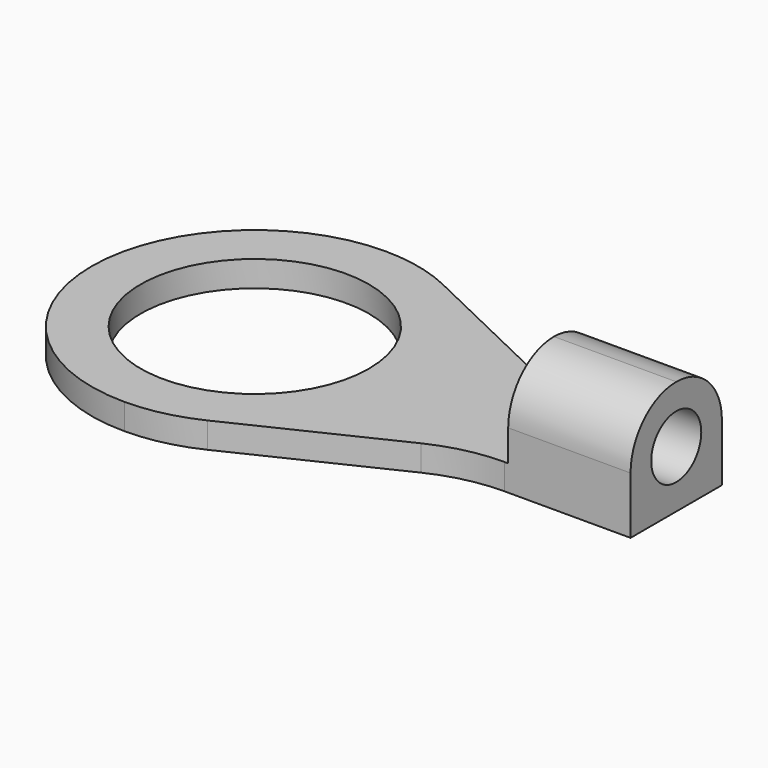
from build123d import *

# Parameters (mm, degrees)
F0_R     = 4.2
F1_DEPTH = 0.95
F2_W     = 4.5
F2_H     = 4.2
F3_DEPTH = 3.25
F4_R     = 2.09999
F5_R     = 1.15
F6_DEPTH = 25


# Not quite as in the source:
# - a fillet or chamfer is up to 0.001 mm smaller than in the source, because OpenCascade refuses the exact size


with BuildPart() as f1:
    # F0 (on Top) → F1 (new body)
    with BuildSketch(Plane.XY):
        with BuildLine():
            Line((16.8637172922, 3.9), (21.5, 3.9))
            Line((21.5, 3.9), (21.5, 8.1))
            Line((21.5, 8.1), (16.8637172922, 8.1))
            ThreePointArc((16.8637172922, 8.1), (15.5339156309, 8.2492199202), (14.2702582689, 8.6894574861))
            Line((14.2702582689, 8.6894574861), (8.5934590232, 11.4105425139))
            ThreePointArc((8.5934590232, 11.4105425139), (7.3298016613, 11.8507800798), (6, 12))
            ThreePointArc((6, 12), (1.7573593129, 10.2426406871), (0, 6))
            ThreePointArc((0, 6), (1.7573593129, 1.7573593129), (6, 0))
            ThreePointArc((6, 0), (7.3298016613, 0.1492199202), (8.5934590232, 0.5894574861))
            Line((8.5934590232, 0.5894574861), (14.2702582689, 3.3105425139))
            ThreePointArc((14.2702582689, 3.3105425139), (15.5339156309, 3.7507800798), (16.8637172922, 3.9))
        make_face()
        with Locations((6, 6)):
            Circle(F0_R, mode=Mode.SUBTRACT)
    extrude(amount=F1_DEPTH)

    # F2 (on face) → F3 (join)
    with BuildSketch(Plane.XY.offset(0.95)):
        with Locations((19.25, 6)):
            Rectangle(F2_W, F2_H)
    extrude(amount=F3_DEPTH)

    # F4 (radius 2.1 in the source; OpenCascade refuses exactly that, so slightly less here)
    f4_edges = [f1.edges().sort_by_distance(p)[0] for p in [
        (19.25, 8.1, 4.2),
        (19.25, 3.9, 4.2),
    ]]
    fillet(f4_edges, radius=F4_R)

    # F5 (on face) → F6 (cut)
    with BuildSketch(Plane.YZ.offset(21.5)):
        with Locations((6, 2.1)):
            Circle(F5_R)
    extrude(amount=-F6_DEPTH, mode=Mode.SUBTRACT)


solid = f1.part
